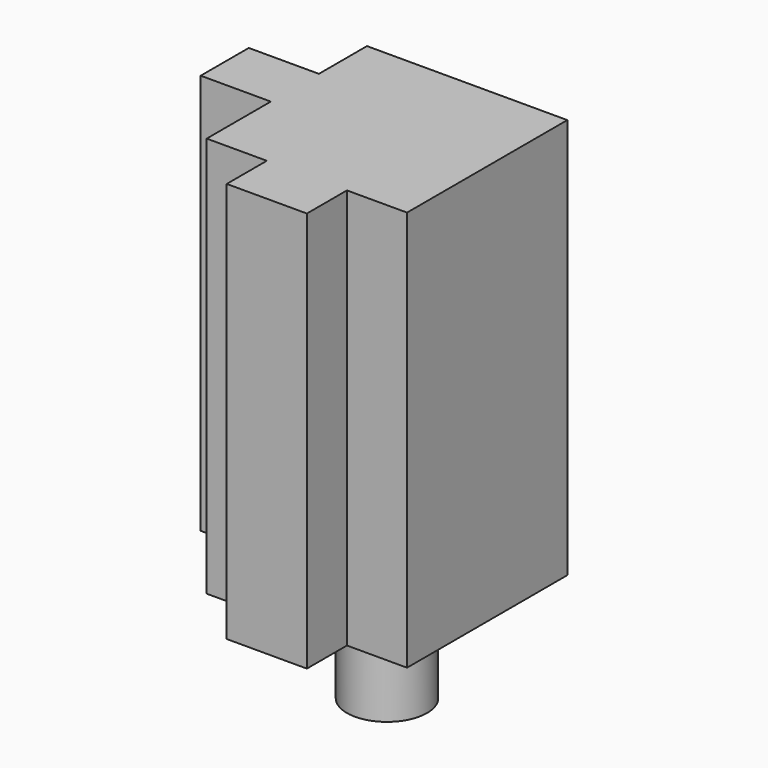
from build123d import *

# Parameters (mm, degrees)
F0_W     = 9.5
F0_H     = 10
F1_DEPTH = 20
F2_W     = 3.5
F2_H     = 3
F3_DEPTH = 20
F2_W_2   = 4
F2_H_2   = 2.5
F5_DEPTH = 20
F6_R     = 2
F7_DEPTH = 5
F8_W     = 10
F8_H     = 20
F9_DEPTH = 0.5


# Not quite as in the source:
# - a feature names something its author has since deleted; it is built from what else it names


with BuildPart() as f1:
    # F0 (on Top) → F1 (new body)
    with BuildSketch(Plane.XY):
        with Locations((4.75, 5)):
            Rectangle(F0_W, F0_H)
    extrude(amount=F1_DEPTH)

    # F2 (on face) → F3 (join, through all)
    with BuildSketch(Plane.XY.offset(20)):
        with Locations((-1.75, 5.5)):
            Rectangle(F2_W, F2_H)
    extrude(amount=-F3_DEPTH)

    # F2 (on face) → F5 (join, through all)
    with BuildSketch(Plane.XY.offset(20)):
        with Locations((5, -1.25)):
            Rectangle(F2_W_2, F2_H_2)
    extrude(amount=-F5_DEPTH)

    # F6 (on face) → F7 (join)
    with BuildSketch(Plane(origin=(0, 0, 0), x_dir=(1, 0, 0), z_dir=(0, 0, -1))):
        with Locations((5, -5)):
            Circle(F6_R)
    extrude(amount=F7_DEPTH)

    # F8 (on face) → F9 (join)
    with BuildSketch(Plane.YZ.offset(9.5)):
        with Locations((5, 10)):
            Rectangle(F8_W, F8_H)
    extrude(amount=F9_DEPTH)


solid = f1.part
